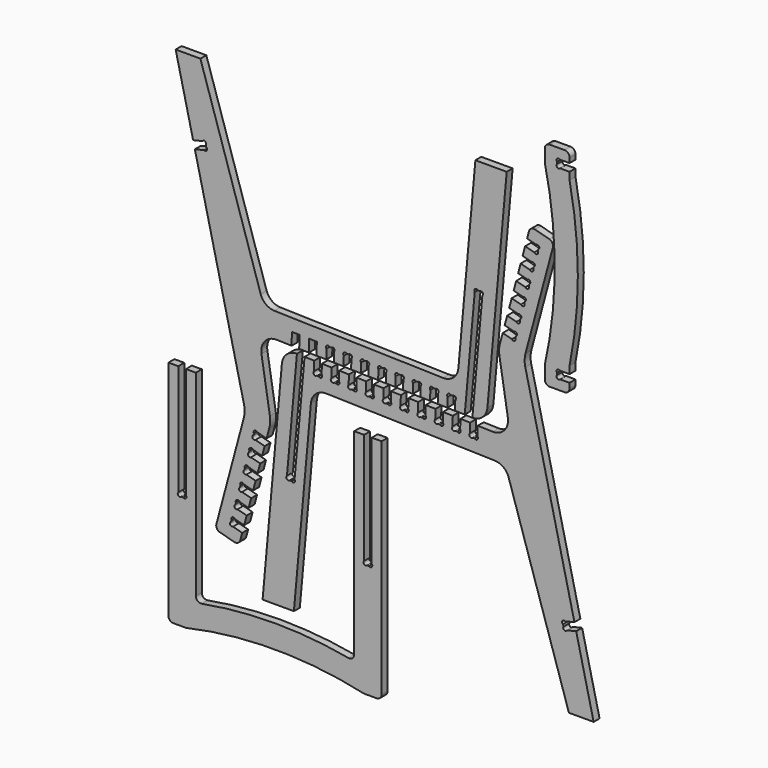
from build123d import *

# Parameters (mm, degrees)
F1_DEPTH = 15


# Not quite as in the source:
# - ends of sketch curves that miss each other by under 0.0002 mm in the source are joined


with BuildPart() as f1:
    # F0 (on Front) → F1 (new body)
    with BuildSketch(Plane.XZ):
        with BuildLine():
            Line((-253.2947544975, 117.7855395442), (-375.1967914229, 497.2499793756))
            Line((-375.1967914229, 497.2499793756), (-425.1905041083, 497.2499793756))
            Line((-425.1905041083, 497.2499793756), (-389.9049438798, 347.4634861898))
            Line((-389.9049438798, 347.4634861898), (-371.079721815, 351.8981891095))
            ThreePointArc((-371.079721815, 351.8981891095), (-365.5742648106, 353.1954035047), (-364.2771991027, 347.6899116411))
            Line((-364.2771991027, 347.6899116411), (-363.3402915905, 343.7127570487))
            ThreePointArc((-363.3402915905, 343.7127570487), (-362.04340432, 338.2073013734), (-367.5488599495, 336.910414392))
            Line((-367.5488599495, 336.910414392), (-386.3742304856, 332.4756771791))
            Line((-386.3742304856, 332.4756771791), (-287.0966620119, -88.9555981658))
            ThreePointArc((-287.0966620119, -88.9555981658), (-285.7704591865, -101.1799567515), (-287.4681614752, -113.3582802867))
            Line((-287.4681614752, -113.3582802867), (-342.8856176788, -320.1790402556))
            ThreePointArc((-342.8856176788, -320.1790402556), (-341.8867385281, -327.7662763407), (-335.8154385368, -332.4249485559))
            Line((-335.8154385368, -332.4249485559), (-306.8413075947, -340.1885438264))
            ThreePointArc((-306.8413075947, -340.1885438264), (-299.2540707132, -339.1896658351), (-294.5953980799, -333.1183650098))
            Line((-294.5953980799, -333.1183650098), (-290.7653584817, -318.8244602709))
            Line((-290.7653584817, -318.8244602709), (-309.4470531415, -313.8187150252))
            ThreePointArc((-309.4470531415, -313.8187150252), (-314.9104678803, -312.3547975138), (-313.4465503383, -306.8913827573))
            Line((-313.4465503383, -306.8913827573), (-312.389072896, -302.9448251785))
            ThreePointArc((-312.389072896, -302.9448251785), (-310.9251553846, -297.4814104398), (-305.4617406281, -298.9453279818))
            Line((-305.4617406281, -298.9453279818), (-286.7800459989, -303.9510732452))
            Line((-286.7800459989, -303.9510732452), (-281.7078303917, -285.0213065398))
            Line((-281.7078303917, -285.0213065398), (-300.3895250515, -280.0155623207))
            ThreePointArc((-300.3895250515, -280.0155623207), (-305.8529397903, -278.5516448093), (-304.3890222483, -273.0882300528))
            Line((-304.3890222483, -273.0882300528), (-303.3315458325, -269.1416714475))
            ThreePointArc((-303.3315458325, -269.1416714475), (-301.8676283211, -263.6782567087), (-296.4042135647, -265.1421742507))
            Line((-296.4042135647, -265.1421742507), (-277.7225189355, -270.1479195141))
            Line((-277.7225189355, -270.1479195141), (-272.6503033283, -251.2181538353))
            Line((-272.6503033283, -251.2181538353), (-291.3319979881, -246.2124085896))
            ThreePointArc((-291.3319979881, -246.2124085896), (-296.7954127269, -244.7484910783), (-295.3314951849, -239.2850763218))
            Line((-295.3314951849, -239.2850763218), (-294.2740177425, -235.338518743))
            ThreePointArc((-294.2740177425, -235.338518743), (-292.8101002312, -229.8751040042), (-287.3466854747, -231.3390215462))
            Line((-287.3466854747, -231.3390215462), (-268.6649908455, -236.3447668096))
            Line((-268.6649908455, -236.3447668096), (-263.5927752383, -217.4150001043))
            Line((-263.5927752383, -217.4150001043), (-282.2744698981, -212.4092558851))
            ThreePointArc((-282.2744698981, -212.4092558851), (-287.7378846369, -210.9453383738), (-286.2739670949, -205.4819236173))
            Line((-286.2739670949, -205.4819236173), (-285.2164906791, -201.535365012))
            ThreePointArc((-285.2164906791, -201.535365012), (-283.7525731677, -196.0719502732), (-278.2891584113, -197.5358678152))
            Line((-278.2891584113, -197.5358678152), (-259.6074627556, -202.5416130786))
            Line((-259.6074627556, -202.5416130786), (-254.5352481749, -183.6118473998))
            Line((-254.5352481749, -183.6118473998), (-273.2169428347, -178.6061021541))
            ThreePointArc((-273.2169428347, -178.6061021541), (-278.6803575735, -177.1421846427), (-277.2164400315, -171.6787698863))
            Line((-277.2164400315, -171.6787698863), (-276.1589625891, -167.7322123075))
            ThreePointArc((-276.1589625891, -167.7322123075), (-274.6950450777, -162.2687975687), (-269.2316303213, -163.7327151107))
            Line((-269.2316303213, -163.7327151107), (-250.5499356921, -168.7384593475))
            Line((-250.5499356921, -168.7384593475), (-245.4777200849, -149.8086936688))
            Line((-245.4777200849, -149.8086936688), (-264.1594147447, -144.8029494496))
            ThreePointArc((-264.1594147447, -144.8029494496), (-269.6228294835, -143.3390319382), (-268.1589119415, -137.8756171818))
            Line((-268.1589119415, -137.8756171818), (-267.1014344992, -133.9290585764))
            ThreePointArc((-267.1014344992, -133.9290585764), (-265.6375182366, -128.4656439659), (-260.1741032578, -129.9295613796))
            Line((-260.1741032578, -129.9295613796), (-241.4924076021, -134.935306643))
            Line((-241.4924076021, -134.935306643), (-235.8021989195, -113.6991584132))
            ThreePointArc((-235.8021989195, -113.6991584132), (-234.1544050353, -103.119134936), (-234.7973871688, -92.4308845484))
            Line((-234.7973871688, -92.4308845484), (-251.8788953518, 12.4408270266))
            ThreePointArc((-251.8788953518, 12.4408270266), (-244.8808698945, 36.9772679339), (-221.5253421179, 47.2499795181))
            Line((-221.5253421179, 47.2499795181), (-190.9510679129, 46.4878614502))
            Line((-190.9510679129, 46.4878614502), (-190.3281713087, 71.4769566858))
            Line((-190.3281713087, 71.4769566858), (-174.9348892187, 71.0932502348))
            Line((-174.9348892187, 71.0932502348), (-175.5577857961, 46.1041560736))
            Line((-175.5577857961, 46.1041560736), (-155.9663355493, 45.6158054559))
            Line((-155.9663355493, 45.6158054559), (-155.3434389731, 70.6048982445))
            Line((-155.3434389731, 70.6048982445), (-139.9501568197, 70.2211956607))
            Line((-139.9501568197, 70.2211956607), (-140.5730534325, 45.2321000793))
            Line((-140.5730534325, 45.2321000793), (-120.9816031857, 44.7437484351))
            Line((-120.9816031857, 44.7437484351), (-120.4996520033, 64.0784564999))
            ThreePointArc((-120.4996520033, 64.0784564999), (-120.3587064075, 69.7328431978), (-114.7043196424, 69.5918975313))
            Line((-114.7043196424, 69.5918975313), (-110.6198108507, 69.4900834136))
            ThreePointArc((-110.6198108507, 69.4900834136), (-104.9654241528, 69.3491378178), (-105.1063698193, 63.6947510526))
            Line((-105.1063698193, 63.6947510526), (-105.588321069, 44.360044085))
            Line((-105.588321069, 44.360044085), (-85.9968708222, 43.8716924408))
            Line((-85.9968708222, 43.8716924408), (-85.5149196398, 63.2064005056))
            ThreePointArc((-85.5149196398, 63.2064005056), (-85.3739740439, 68.8607872035), (-79.7195872788, 68.719841537))
            Line((-79.7195872788, 68.719841537), (-75.6350784871, 68.6180274193))
            ThreePointArc((-75.6350784871, 68.6180274193), (-69.9806917892, 68.4770818235), (-70.1216374557, 62.8226950583))
            Line((-70.1216374557, 62.8226950583), (-70.6035887054, 43.4879870642))
            Line((-70.6035887054, 43.4879870642), (-51.0121384586, 42.9996354199))
            Line((-51.0121384586, 42.9996354199), (-50.5301872762, 62.3343434848))
            ThreePointArc((-50.5301872762, 62.3343434848), (-50.3892416804, 67.9887301827), (-44.7348549152, 67.8477845162))
            Line((-44.7348549152, 67.8477845162), (-40.6503461235, 67.745971425))
            ThreePointArc((-40.6503461235, 67.745971425), (-34.9959594256, 67.6050258292), (-35.1369050921, 61.950639064))
            Line((-35.1369050921, 61.950639064), (-35.6188563418, 42.6159310699))
            Line((-35.6188563418, 42.6159310699), (-16.0274071216, 42.1275794256))
            Line((-16.0274071216, 42.1275794256), (-15.5454549126, 61.4622874905))
            ThreePointArc((-15.5454549126, 61.4622874905), (-15.4045093168, 67.1166741884), (-9.7501225516, 66.9757285219))
            Line((-9.7501225516, 66.9757285219), (-5.6656137599, 66.8739144042))
            ThreePointArc((-5.6656137599, 66.8739144042), (-0.011227062, 66.7329688084), (-0.1521727286, 61.0785820432))
            Line((-0.1521727286, 61.0785820432), (-0.6341239782, 41.743874049))
            Line((-0.6341239782, 41.743874049), (18.957325242, 41.2555234313))
            Line((18.957325242, 41.2555234313), (19.439277451, 60.5902304697))
            ThreePointArc((19.439277451, 60.5902304697), (19.5802230468, 66.2446171676), (25.2346098119, 66.1036715011))
            Line((25.2346098119, 66.1036715011), (29.3191186036, 66.0018584099))
            ThreePointArc((29.3191186036, 66.0018584099), (34.9735053015, 65.8609128141), (34.832559635, 60.2065260489))
            Line((34.832559635, 60.2065260489), (34.3506073588, 40.8718180547))
            Line((34.3506073588, 40.8718180547), (53.9420576056, 40.3834664105))
            Line((53.9420576056, 40.3834664105), (54.4240098145, 59.7181744754))
            ThreePointArc((54.4240098145, 59.7181744754), (54.5649554104, 65.3725611733), (60.2193421755, 65.2316155068))
            Line((60.2193421755, 65.2316155068), (64.3038509672, 65.129801389))
            ThreePointArc((64.3038509672, 65.129801389), (69.9582376651, 64.9888557932), (69.8172919986, 59.3344690281))
            Line((69.8172919986, 59.3344690281), (69.3353397224, 39.9997620605))
            Line((69.3353397224, 39.9997620605), (88.9267899692, 39.5114104162))
            Line((88.9267899692, 39.5114104162), (89.4087421781, 58.8461184811))
            ThreePointArc((89.4087421781, 58.8461184811), (89.5496877739, 64.500505179), (95.2040745391, 64.3595595125))
            Line((95.2040745391, 64.3595595125), (99.2885833308, 64.2577453948))
            ThreePointArc((99.2885833308, 64.2577453948), (104.9429700287, 64.1167997989), (104.8020243622, 58.4624130338))
            Line((104.8020243622, 58.4624130338), (104.320072086, 39.1277050396))
            Line((104.320072086, 39.1277050396), (123.9115223327, 38.6393533954))
            Line((123.9115223327, 38.6393533954), (124.3934745417, 57.9740614602))
            ThreePointArc((124.3934745417, 57.9740614602), (124.5344201375, 63.6284481581), (130.1888069027, 63.4875024916))
            Line((130.1888069027, 63.4875024916), (134.2733156944, 63.3856894005))
            ThreePointArc((134.2733156944, 63.3856894005), (139.9277023923, 63.2447438046), (139.7867567257, 57.5903570395))
            Line((139.7867567257, 57.5903570395), (139.3048044495, 38.2556490453))
            Line((139.3048044495, 38.2556490453), (158.8799768899, 37.7677028834))
            Line((158.8799768899, 37.7677028834), (179.127410315, 262.3772033679))
            ThreePointArc((179.127410315, 262.3772033679), (179.6352233392, 268.0105046787), (185.2685248328, 267.5026903073))
            Line((185.2685248328, 267.5026903073), (189.3378027282, 267.1358651237))
            ThreePointArc((189.3378027282, 267.1358651237), (194.9711032233, 266.6280508205), (194.4632892462, 260.9947500844))
            Line((194.4632892462, 260.9947500844), (174.3058854506, 37.3839646576))
            ThreePointArc((174.3058854506, 37.3839646576), (194.8762338774, 45.0549412897), (204.7121902621, 64.6823983409))
            Line((204.7121902621, 64.6823983409), (243.7060139572, 497.2499793756))
            Line((243.7060139572, 497.2499793756), (180.4381304549, 497.2499793756))
            Line((180.4381304549, 497.2499793756), (146.0841315247, 116.1530491461))
            ThreePointArc((146.0841315247, 116.1530491461), (136.1675653992, 96.4534837558), (115.4615659045, 88.8592265136))
            Line((115.4615659045, 88.8592265136), (-225.6110253428, 97.3610653416))
            ThreePointArc((-225.6110253428, 97.3610653416), (-242.6719362321, 103.210144471), (-253.2947544975, 117.7855395442))
        make_face()
    extrude(amount=F1_DEPTH)


with BuildPart() as f1b:
    # F0 (on Front) → F1, piece 2 (new body)
    with BuildSketch(Plane.XZ):
        with BuildLine():
            Line((247.4616930625, -44.6801124798), (369.3637299879, -424.1445523112))
            Line((369.3637299879, -424.1445523112), (419.3574426734, -424.1445523112))
            Line((419.3574426734, -424.1445523112), (384.0718824449, -274.3580591254))
            Line((384.0718824449, -274.3580591254), (365.24666038, -278.792762045))
            ThreePointArc((365.24666038, -278.792762045), (359.7412033756, -280.0899764403), (358.4441376677, -274.5844845767))
            Line((358.4441376677, -274.5844845767), (357.5072301556, -270.6073299843))
            ThreePointArc((357.5072301556, -270.6073299843), (356.210342885, -265.1018743089), (361.7157985145, -263.8049873276))
            Line((361.7157985145, -263.8049873276), (380.5411690506, -259.3702501146))
            Line((380.5411690506, -259.3702501146), (281.2636005769, 162.0610252302))
            ThreePointArc((281.2636005769, 162.0610252302), (279.937397744, 174.2853833203), (281.6350997836, 186.4637063934))
            Line((281.6350997836, 186.4637063934), (337.0525562438, 393.28446732))
            ThreePointArc((337.0525562438, 393.28446732), (336.0536770931, 400.8717034051), (329.9823771018, 405.5303756204))
            Line((329.9823771018, 405.5303756204), (301.0082461597, 413.2939708909))
            ThreePointArc((301.0082461597, 413.2939708909), (293.4210094774, 412.2950919881), (288.7623368328, 406.2237917488))
            Line((288.7623368328, 406.2237917488), (284.9322970467, 391.9298873353))
            Line((284.9322970467, 391.9298873353), (303.6139917065, 386.9241420896))
            ThreePointArc((303.6139917065, 386.9241420896), (309.0774064453, 385.4602245783), (307.6134889033, 379.9968098218))
            Line((307.6134889033, 379.9968098218), (306.556011461, 376.050252243))
            ThreePointArc((306.556011461, 376.050252243), (305.0920939496, 370.5868375042), (299.6286791931, 372.0507550462))
            Line((299.6286791931, 372.0507550462), (280.946984564, 377.0564992831))
            Line((280.946984564, 377.0564992831), (275.8747689568, 358.1267336043))
            Line((275.8747689568, 358.1267336043), (294.5564636166, 353.1209893851))
            ThreePointArc((294.5564636166, 353.1209893851), (300.0198783553, 351.6570718738), (298.5559608133, 346.1936571173))
            Line((298.5559608133, 346.1936571173), (297.4984843975, 342.2470985119))
            ThreePointArc((297.4984843975, 342.2470985119), (296.0345668862, 336.7836837732), (290.5711521297, 338.2476013152))
            Line((290.5711521297, 338.2476013152), (271.889456474, 343.2533465786))
            Line((271.889456474, 343.2533465786), (266.8172418933, 324.3235808998))
            Line((266.8172418933, 324.3235808998), (285.4989365531, 319.3178356541))
            ThreePointArc((285.4989365531, 319.3178356541), (290.9623512919, 317.8539181427), (289.4984337499, 312.3905033863))
            Line((289.4984337499, 312.3905033863), (288.4409563076, 308.4439458074))
            ThreePointArc((288.4409563076, 308.4439458074), (286.9770387962, 302.9805310687), (281.5136240397, 304.4444486107))
            Line((281.5136240397, 304.4444486107), (262.8319294106, 309.4501928475))
            Line((262.8319294106, 309.4501928475), (257.7597138034, 290.5204271688))
            Line((257.7597138034, 290.5204271688), (276.4414084631, 285.5146819231))
            ThreePointArc((276.4414084631, 285.5146819231), (281.9048230736, 284.0507656605), (280.4409056599, 278.5873506818))
            Line((280.4409056599, 278.5873506818), (279.3834282176, 274.6407920764))
            ThreePointArc((279.3834282176, 274.6407920764), (277.919511955, 269.1773774659), (272.4560969763, 270.6412948796))
            Line((272.4560969763, 270.6412948796), (253.7744013206, 275.647040143))
            Line((253.7744013206, 275.647040143), (248.7021867399, 256.7172744642))
            Line((248.7021867399, 256.7172744642), (267.3838813997, 251.7115292186))
            ThreePointArc((267.3838813997, 251.7115292186), (272.8472961385, 250.2476117072), (271.3833785965, 244.7841969507))
            Line((271.3833785965, 244.7841969507), (270.3259011541, 240.8376383454))
            ThreePointArc((270.3259011541, 240.8376383454), (268.8619832578, 235.3742233843), (263.3985684418, 236.8381419185))
            Line((263.3985684418, 236.8381419185), (244.7168742571, 241.843886412))
            Line((244.7168742571, 241.843886412), (239.6446586499, 222.9141207332))
            Line((239.6446586499, 222.9141207332), (258.3263533097, 217.9083754875))
            ThreePointArc((258.3263533097, 217.9083754875), (263.7897679202, 216.4444581984), (262.325850951, 210.9810434763))
            Line((262.325850951, 210.9810434763), (261.2683730642, 207.0344856409))
            ThreePointArc((261.2683730642, 207.0344856409), (259.804455775, 201.5710710304), (254.341041053, 203.0349879996))
            Line((254.341041053, 203.0349879996), (235.6593461672, 208.0407337075))
            Line((235.6593461672, 208.0407337075), (229.9691374845, 186.8045844511))
            ThreePointArc((229.9691374845, 186.8045844511), (228.3213435769, 176.2245615052), (228.9643257338, 165.5363116129))
            Line((228.9643257338, 165.5363116129), (246.0458339168, 60.6645990113))
            ThreePointArc((246.0458339168, 60.6645990113), (239.0478081265, 36.1281587488), (215.6922806829, 25.8554475464))
            Line((215.6922806829, 25.8554475464), (185.1180064779, 26.6175656143))
            Line((185.1180064779, 26.6175656143), (184.6360552955, 7.2828575494))
            ThreePointArc((184.6360552955, 7.2828575494), (184.4951096997, 1.6284708515), (178.8407229345, 1.769416518))
            Line((178.8407229345, 1.769416518), (174.7562141428, 1.8712306357))
            ThreePointArc((174.7562141428, 1.8712306357), (169.1018266747, 2.0121759621), (169.2427720849, 7.6665629967))
            Line((169.2427720849, 7.6665629967), (169.7247243611, 27.0012699643))
            Line((169.7247243611, 27.0012699643), (150.1332741143, 27.4896216086))
            Line((150.1332741143, 27.4896216086), (149.6513229319, 8.1549145702))
            ThreePointArc((149.6513229319, 8.1549145702), (149.5103776055, 2.5005281286), (143.8559910836, 2.641473))
            Line((143.8559910836, 2.641473), (139.7714817793, 2.74328663))
            ThreePointArc((139.7714817793, 2.74328663), (134.1170950814, 2.8842322258), (134.2580407479, 8.538618991))
            Line((134.2580407479, 8.538618991), (134.7399919975, 27.8733269852))
            Line((134.7399919975, 27.8733269852), (115.1485417508, 28.3616786294))
            Line((115.1485417508, 28.3616786294), (114.6665905683, 9.0269705645))
            ThreePointArc((114.6665905683, 9.0269705645), (114.5256449725, 3.3725838666), (108.8712582074, 3.5135295331))
            Line((108.8712582074, 3.5135295331), (104.7867494157, 3.6153426243))
            ThreePointArc((104.7867494157, 3.6153426243), (99.1323627178, 3.7562882201), (99.2733083843, 9.4106749853))
            Line((99.2733083843, 9.4106749853), (99.755259634, 28.7453829794))
            Line((99.755259634, 28.7453829794), (80.1638093872, 29.2337346237))
            Line((80.1638093872, 29.2337346237), (79.6818582048, 9.8990265588))
            ThreePointArc((79.6818582048, 9.8990265588), (79.540912609, 4.2446398609), (73.8865258438, 4.3855855274))
            Line((73.8865258438, 4.3855855274), (69.8020170521, 4.4873996451))
            ThreePointArc((69.8020170521, 4.4873996451), (64.1476303542, 4.628345241), (64.2885760207, 10.2827320061))
            Line((64.2885760207, 10.2827320061), (64.7705272704, 29.6174400003))
            Line((64.7705272704, 29.6174400003), (45.1790770236, 30.1057916445))
            Line((45.1790770236, 30.1057916445), (44.6971258412, 10.7710835797))
            ThreePointArc((44.6971258412, 10.7710835797), (44.5561802454, 5.1166968818), (38.9017934802, 5.2576425483))
            Line((38.9017934802, 5.2576425483), (34.8172846885, 5.3594556394))
            ThreePointArc((34.8172846885, 5.3594556394), (29.1628979906, 5.5004012353), (29.3038436572, 11.1547880004))
            Line((29.3038436572, 11.1547880004), (29.7857949068, 30.4894959946))
            Line((29.7857949068, 30.4894959946), (10.1943456866, 30.9778476388))
            Line((10.1943456866, 30.9778476388), (9.7123934776, 11.6431395739))
            ThreePointArc((9.7123934776, 11.6431395739), (9.5714478818, 5.988752876), (3.9170611167, 6.1296985426))
            Line((3.9170611167, 6.1296985426), (-0.167447675, 6.2315126603))
            ThreePointArc((-0.167447675, 6.2315126603), (-5.8218343729, 6.3724582561), (-5.6808887064, 12.0268450212))
            Line((-5.6808887064, 12.0268450212), (-5.1989374567, 31.3615519889))
            Line((-5.1989374567, 31.3615519889), (-24.790386677, 31.8499036331))
            Line((-24.790386677, 31.8499036331), (-25.2723388859, 12.5151965948))
            ThreePointArc((-25.2723388859, 12.5151965948), (-25.4132844818, 6.8608098969), (-31.0676712469, 7.0017555634))
            Line((-31.0676712469, 7.0017555634), (-35.1521800386, 7.1035686546))
            ThreePointArc((-35.1521800386, 7.1035686546), (-40.8065667365, 7.2445142504), (-40.66562107, 12.8989010155))
            Line((-40.66562107, 12.8989010155), (-40.1836698203, 32.2336090097))
            Line((-40.1836698203, 32.2336090097), (-59.7751190406, 32.7219606539))
            Line((-59.7751190406, 32.7219606539), (-60.2570712495, 13.3872525891))
            ThreePointArc((-60.2570712495, 13.3872525891), (-60.3980168453, 7.7328658912), (-66.0524036105, 7.8738115577))
            Line((-66.0524036105, 7.8738115577), (-70.1369124022, 7.9756246489))
            ThreePointArc((-70.1369124022, 7.9756246489), (-75.7912991001, 8.1165702447), (-75.6503534336, 13.7709570098))
            Line((-75.6503534336, 13.7709570098), (-75.1684011574, 33.105665004))
            Line((-75.1684011574, 33.105665004), (-94.7598514041, 33.5940166482))
            Line((-94.7598514041, 33.5940166482), (-95.2418036131, 14.2593085834))
            ThreePointArc((-95.2418036131, 14.2593085834), (-95.3827492089, 8.6049218855), (-101.0371359741, 8.745867552))
            Line((-101.0371359741, 8.745867552), (-105.1216447658, 8.8476816697))
            ThreePointArc((-105.1216447658, 8.8476816697), (-110.7760314637, 8.9886272655), (-110.6350857971, 14.6430140307))
            Line((-110.6350857971, 14.6430140307), (-110.1531335209, 33.9777220248))
            Line((-110.1531335209, 33.9777220248), (-129.7445837677, 34.4660736691))
            Line((-129.7445837677, 34.4660736691), (-130.2265359767, 15.1313656042))
            ThreePointArc((-130.2265359767, 15.1313656042), (-130.3674815725, 9.4769789063), (-136.0218683376, 9.6179245728))
            Line((-136.0218683376, 9.6179245728), (-140.1063771293, 9.719737664))
            ThreePointArc((-140.1063771293, 9.719737664), (-145.7607638272, 9.8606832598), (-145.6198181607, 15.515070025))
            Line((-145.6198181607, 15.515070025), (-145.1378658845, 34.8497780191))
            Line((-145.1378658845, 34.8497780191), (-164.7130383249, 35.337724181))
            Line((-164.7130383249, 35.337724181), (-184.9604717499, -189.2717763034))
            ThreePointArc((-184.9604717499, -189.2717763034), (-185.4682847742, -194.9050776143), (-191.1015862678, -194.3972632429))
            Line((-191.1015862678, -194.3972632429), (-195.1708641632, -194.0304380593))
            ThreePointArc((-195.1708641632, -194.0304380593), (-200.8041646583, -193.522623756), (-200.2963506812, -187.8893230199))
            Line((-200.2963506812, -187.8893230199), (-180.1389468856, 35.7214613803))
            ThreePointArc((-180.1389468856, 35.7214613803), (-200.7092953056, 28.0504857808), (-210.545251697, 8.4230287236))
            Line((-210.545251697, 8.4230287236), (-249.5390753921, -424.1445523112))
            Line((-249.5390753921, -424.1445523112), (-186.2711918899, -424.1445523112))
            Line((-186.2711918899, -424.1445523112), (-151.9171929597, -43.0476220817))
            ThreePointArc((-151.9171929597, -43.0476220817), (-142.0006268342, -23.3480566914), (-121.2946273395, -15.7537994492))
            Line((-121.2946273395, -15.7537994492), (219.7779639079, -24.2556382772))
            ThreePointArc((219.7779639079, -24.2556382772), (236.8388747971, -30.1047174065), (247.4616930625, -44.6801124798))
        make_face()
    extrude(amount=F1_DEPTH)


with BuildPart() as f1c:
    # F0 (on Front) → F1, piece 3 (new body)
    with BuildSketch(Plane.XZ):
        with BuildLine():
            Line((-9.052715573, -514.6991269213), (-9.052715573, -64.3209515027))
            Line((-9.052715573, -64.3209515027), (-29.0502014684, -64.3209515027))
            Line((-29.0502014684, -64.3209515027), (-29.0502014684, -288.8532676529))
            ThreePointArc((-29.0502014684, -288.8532676529), (-29.0502011516, -294.5094104894), (-34.7063445616, -294.5094097195))
            Line((-34.7063445616, -294.5094097195), (-38.7921221642, -294.5094096593))
            ThreePointArc((-38.7921221642, -294.5094096593), (-44.4482644875, -294.5094104894), (-44.4482652574, -288.8532675927))
            Line((-44.4482652574, -288.8532675927), (-44.4482651972, -64.3209515027))
            Line((-44.4482651972, -64.3209515027), (-64.4457500661, -64.3209515027))
            Line((-64.4457500661, -64.3209515027), (-64.4457500661, -461.6066555377))
            ThreePointArc((-64.4457500661, -461.6066555377), (-68.0452522941, -469.289401059), (-76.2521499413, -471.4406393168))
            ThreePointArc((-76.2521499413, -471.4406393168), (-224.4256331232, -457.9353455032), (-372.5991163724, -471.4406389501))
            ThreePointArc((-372.5991163724, -471.4406389501), (-380.8060139523, -469.289401059), (-384.4055161802, -461.6066555377))
            Line((-384.4055161802, -461.6066555377), (-384.4055161802, -64.3209515027))
            Line((-384.4055161802, -64.3209515027), (-404.4030010491, -64.3209515027))
            Line((-404.4030010491, -64.3209515027), (-404.4030010491, -288.8532676529))
            ThreePointArc((-404.4030010491, -288.8532676529), (-404.4030017588, -294.5094104894), (-410.0591446555, -294.5094102328))
            Line((-410.0591446555, -294.5094102328), (-414.144921745, -294.5094096593))
            ThreePointArc((-414.144921745, -294.5094096593), (-419.8010650948, -294.5094104894), (-419.8010653514, -288.8532670794))
            Line((-419.8010653514, -288.8532670794), (-419.801064778, -64.3209515027))
            Line((-419.801064778, -64.3209515027), (-439.7985506734, -64.3209515027))
            Line((-439.7985506734, -64.3209515027), (-439.7985506734, -514.6991269213))
            ThreePointArc((-439.7985506734, -514.6991269213), (-436.8699866673, -521.769305863), (-429.7998077257, -524.697869869))
            Line((-429.7998077257, -524.697869869), (-404.3696816923, -524.6978688425))
            ThreePointArc((-404.3696816923, -524.6978688425), (-224.4256331232, -504.7003624164), (-44.481584655, -524.6978692909))
            Line((-44.481584655, -524.6978692909), (-19.0514585207, -524.6978688425))
            ThreePointArc((-19.0514585207, -524.6978688425), (-11.981279579, -521.769305863), (-9.052715573, -514.6991269213))
        make_face()
    extrude(amount=F1_DEPTH)


with BuildPart() as f1d:
    # F0 (on Front) → F1, piece 4 (new body)
    with BuildSketch(Plane.XZ):
        with BuildLine():
            ThreePointArc((320.6760220575, 538.5075730069), (340.6735289815, 358.5635243189), (320.6760220575, 178.6194756308))
            Line((320.6760220575, 178.6194756308), (320.6760215288, 153.1893497164))
            ThreePointArc((320.6760215288, 153.1893497164), (323.6045855348, 146.1191707747), (330.6747644765, 143.1906067687))
            Line((330.6747644765, 143.1906067687), (360.663493436, 143.1906067687))
            ThreePointArc((360.663493436, 143.1906067687), (367.7336723777, 146.1191707747), (370.6622363837, 153.1893497164))
            Line((370.6622363837, 153.1893497164), (370.6622363837, 163.1880926641))
            Line((370.6622363837, 163.1880926641), (351.3215220475, 163.1880926641))
            ThreePointArc((351.3215220475, 163.1880926641), (345.6653794676, 163.1880920907), (345.6653794676, 168.844235244))
            Line((345.6653794676, 168.844235244), (345.6653790145, 172.9300133599))
            ThreePointArc((345.6653790145, 172.9300133599), (345.6653794676, 178.5861559398), (351.3215221076, 178.5861564531))
            Line((351.3215221076, 178.5861564531), (370.6622363837, 178.5861563929))
            Line((370.6622363837, 178.5861563929), (370.6622363837, 193.5842708145))
            ThreePointArc((370.6622363837, 193.5842708145), (387.4385458947, 358.5635248216), (370.6622362077, 523.5427788136))
            Line((370.6622362077, 523.5427788136), (370.6622363837, 538.5408932713))
            Line((370.6622363837, 538.5408932713), (351.3215220475, 538.5408932713))
            ThreePointArc((351.3215220475, 538.5408932713), (345.6653794676, 538.5408926979), (345.6653794676, 544.1970358512))
            Line((345.6653794676, 544.1970358512), (345.6653790145, 548.2828139672))
            ThreePointArc((345.6653790145, 548.2828139672), (345.6653794676, 553.9389565471), (351.3215221076, 553.9389570603))
            Line((351.3215221076, 553.9389570603), (370.6622363837, 553.9389570002))
            Line((370.6622363837, 553.9389570002), (370.6622363837, 563.9376989213))
            ThreePointArc((370.6622363837, 563.9376989213), (367.7336723777, 571.007877863), (360.663493436, 573.936441869))
            Line((360.663493436, 573.936441869), (330.6747644765, 573.936441869))
            ThreePointArc((330.6747644765, 573.936441869), (323.6045855348, 571.007877863), (320.6760215288, 563.9376989213))
            Line((320.6760215288, 563.9376989213), (320.6760220575, 538.5075730069))
        make_face()
    extrude(amount=F1_DEPTH)


solid = Compound([f1.part, f1b.part, f1c.part, f1d.part])
